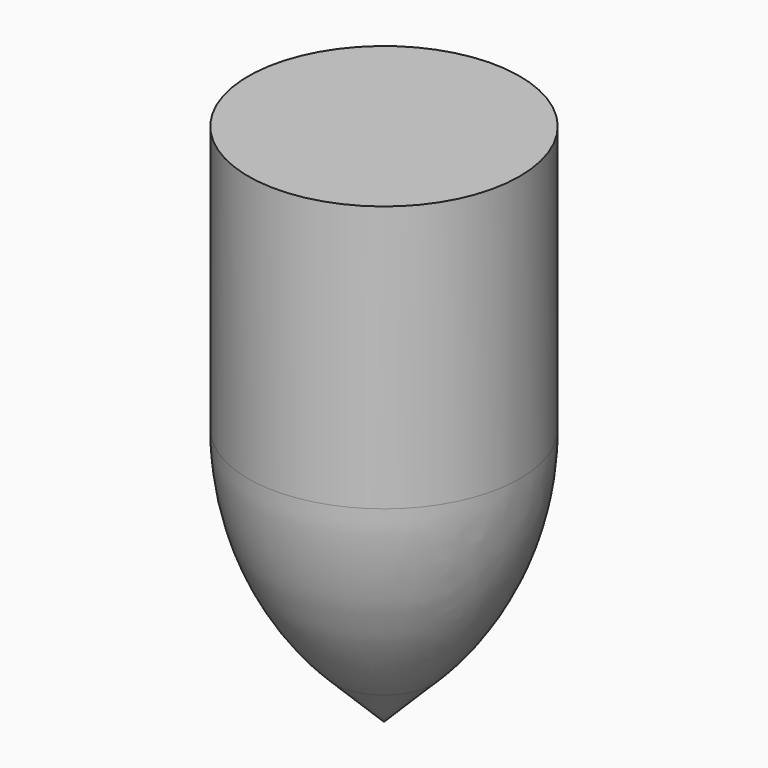
from build123d import *

# Parameters (mm, degrees)
F1_R     = 16.3135462342
F2_DEPTH = 46.736
F4_R     = 35.56


# Not quite as in the source:
# - an extrude whose draft closes it to a point is written as a loft to that point


with BuildPart() as f2:
    # F1 (on face) → F2 (new body)
    with BuildSketch(Plane.XY):
        Circle(F1_R)
    extrude(amount=F2_DEPTH)

    # F1 (on face) → F3 section 0
    with BuildSketch(Plane.XY, mode=Mode.PRIVATE) as f3_s0:
        Circle(F1_R)
    loft([f3_s0.sketch, Vertex(0, 0, -16.3135462342)], ruled=True)

    # F4
    f4_edges = [f2.edges().sort_by_distance(p)[0] for p in [
        (-16.313546, 0, 0),
    ]]
    fillet(f4_edges, radius=F4_R)


solid = f2.part
